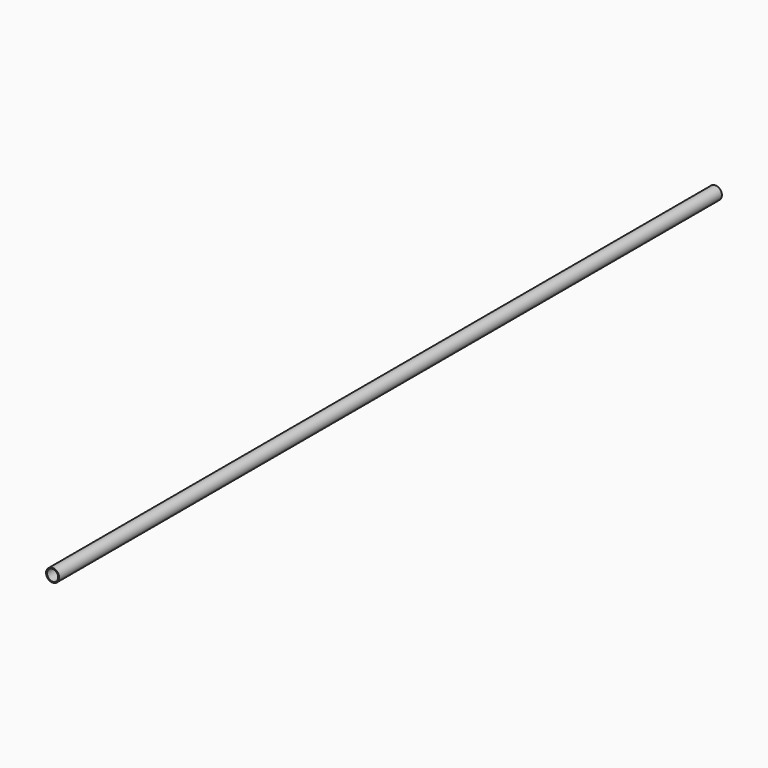
from build123d import *

# Parameters (mm, degrees)
F0_R     = 2.14249
F1_DEPTH = 271.526
F2_R     = 1.8383366591
F3_DEPTH = 12.7


# Not quite as in the source:
# - the program builds the solid bodies; features that only make, move or delete a surface that nothing else refers to are left out


with BuildPart() as f1:
    # F0 (on Front) → F1 (new body)
    with BuildSketch(Plane.XZ):
        with Locations((16.5096987039, -18.3188896626)):
            Circle(F0_R)
    extrude(amount=F1_DEPTH)

    # F2 (on face) → F3 (cut)
    with BuildSketch(Plane.XZ.offset(271.526)):
        with Locations((16.5096987039, -18.3188896626)):
            Circle(F2_R)
    extrude(amount=-F3_DEPTH, mode=Mode.SUBTRACT)


solid = f1.part
